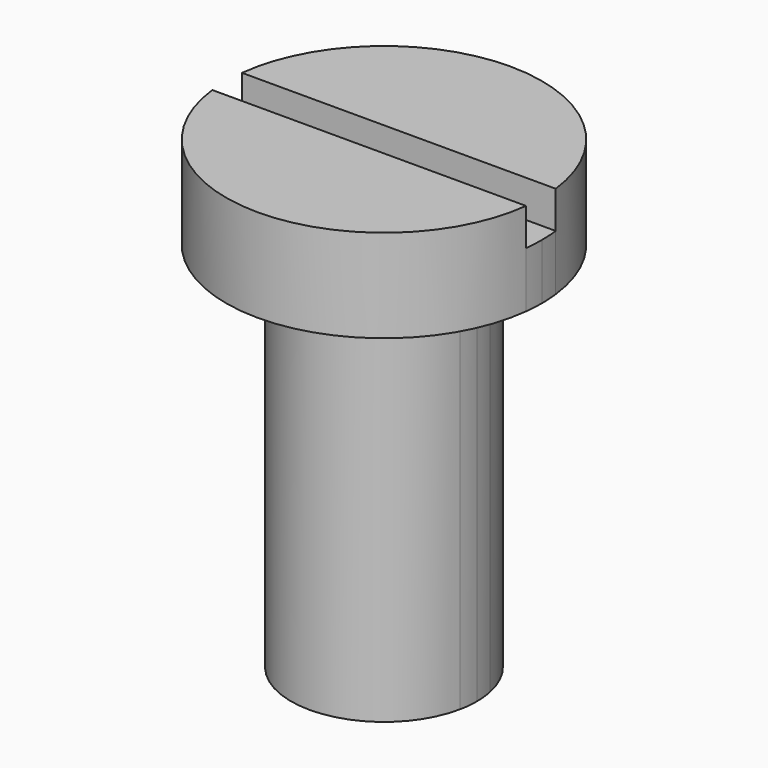
from build123d import *

# Parameters (mm, degrees)
F1_DEPTH = 10
F2_DEPTH = 2.5
F3_DEPTH = 1.5


# Not quite as in the source:
# - a feature names something its author has since deleted; it is built from what else it names


with BuildPart() as f1:
    # F0 (on Top) → F1 (new body)
    with BuildSketch(Plane.XY):
        with BuildLine():
            Line((-2.4494897428, 0.5), (2.4494897428, 0.5))
            ThreePointArc((2.4494897428, 0.5), (0, 2.5), (-2.4494897428, 0.5))
        make_face()
        with BuildLine():
            ThreePointArc((2.5, 0), (2.4873403825, 0.251272405), (2.4494897428, 0.5))
            Line((2.4494897428, 0.5), (-2.4494897428, 0.5))
            ThreePointArc((-2.4494897428, 0.5), (-2.5, 0), (-2.4494897428, -0.5))
            Line((-2.4494897428, -0.5), (2.4494897428, -0.5))
            ThreePointArc((2.4494897428, -0.5), (2.4873403825, -0.251272405), (2.5, 0))
        make_face()
        with BuildLine():
            ThreePointArc((-2.4494897428, -0.5), (0, -2.5), (2.4494897428, -0.5))
            Line((2.4494897428, -0.5), (-2.4494897428, -0.5))
        make_face()
    extrude(amount=-F1_DEPTH)

    # F0 (on Top) → F2 (join)
    with BuildSketch(Plane.XY):
        with BuildLine():
            ThreePointArc((-4.220485754, -0.5), (0, -4.25), (4.220485754, -0.5))
            Line((4.220485754, -0.5), (2.4494897428, -0.5))
            ThreePointArc((2.4494897428, -0.5), (0, -2.5), (-2.4494897428, -0.5))
            Line((-2.4494897428, -0.5), (-4.220485754, -0.5))
        make_face()
        with BuildLine():
            Line((2.4494897428, 0.5), (4.220485754, 0.5))
            ThreePointArc((4.220485754, 0.5), (0, 4.25), (-4.220485754, 0.5))
            Line((-4.220485754, 0.5), (-2.4494897428, 0.5))
            ThreePointArc((-2.4494897428, 0.5), (0, 2.5), (2.4494897428, 0.5))
        make_face()
        with BuildLine():
            Line((-2.4494897428, 0.5), (2.4494897428, 0.5))
            ThreePointArc((2.4494897428, 0.5), (0, 2.5), (-2.4494897428, 0.5))
        make_face()
        with BuildLine():
            ThreePointArc((-2.4494897428, -0.5), (0, -2.5), (2.4494897428, -0.5))
            Line((2.4494897428, -0.5), (-2.4494897428, -0.5))
        make_face()
    extrude(amount=F2_DEPTH)

    # F0 (on Top) → F3 (join)
    with BuildSketch(Plane.XY):
        with BuildLine():
            Line((-2.4494897428, 0.5), (-4.220485754, 0.5))
            ThreePointArc((-4.220485754, 0.5), (-4.25, 0), (-4.220485754, -0.5))
            Line((-4.220485754, -0.5), (-2.4494897428, -0.5))
            ThreePointArc((-2.4494897428, -0.5), (-2.5, 0), (-2.4494897428, 0.5))
        make_face()
        with BuildLine():
            ThreePointArc((2.5, 0), (2.4873403825, 0.251272405), (2.4494897428, 0.5))
            Line((2.4494897428, 0.5), (-2.4494897428, 0.5))
            ThreePointArc((-2.4494897428, 0.5), (-2.5, 0), (-2.4494897428, -0.5))
            Line((-2.4494897428, -0.5), (2.4494897428, -0.5))
            ThreePointArc((2.4494897428, -0.5), (2.4873403825, -0.251272405), (2.5, 0))
        make_face()
        with BuildLine():
            ThreePointArc((4.220485754, -0.5), (4.2426150223, -0.2504351666), (4.25, 0))
            ThreePointArc((4.25, 0), (4.2426150223, 0.2504351666), (4.220485754, 0.5))
            Line((4.220485754, 0.5), (2.4494897428, 0.5))
            ThreePointArc((2.4494897428, 0.5), (2.4873403825, 0.251272405), (2.5, 0))
            ThreePointArc((2.5, 0), (2.4873403825, -0.251272405), (2.4494897428, -0.5))
            Line((2.4494897428, -0.5), (4.220485754, -0.5))
        make_face()
    extrude(amount=F3_DEPTH)


solid = f1.part
